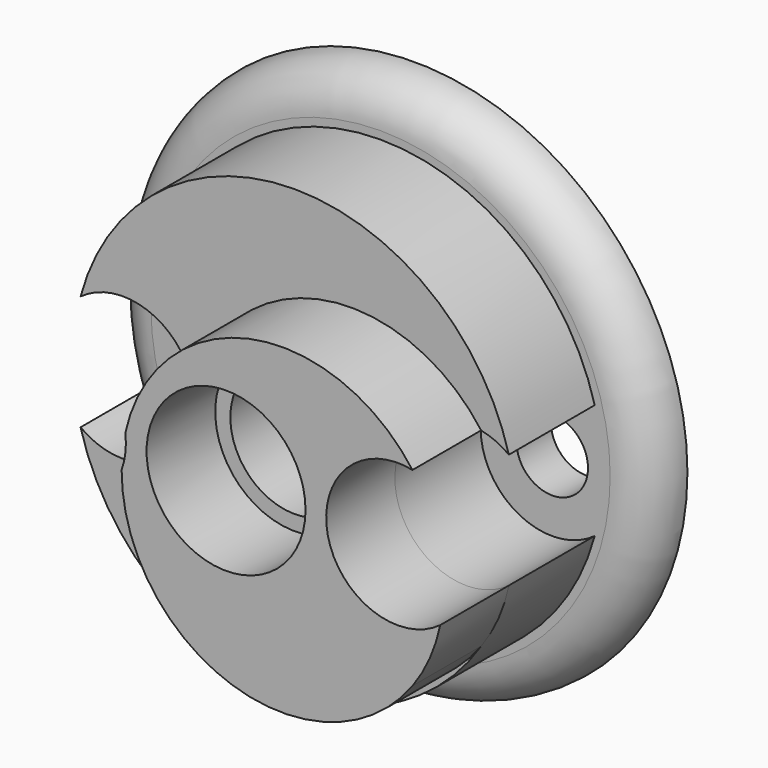
from build123d import *

# Parameters (mm, degrees)
F0_R     = 19.05
F0_R_2   = 2.5
F0_R_3   = 4.5
F1_DEPTH = 3
F2_R     = 2.99999
F3_R     = 4.5
F4_DEPTH = 7.5
F5_R     = 5.555
F6_DEPTH = 6


# Not quite as in the source:
# - a fillet or chamfer is up to 0.001 mm smaller than in the source, because OpenCascade refuses the exact size


with BuildPart() as f1:
    # F0 (on Front) → F1 (new body)
    with BuildSketch(Plane.XZ):
        Circle(F0_R)
        with Locations((-12, 0)):
            Circle(F0_R_2, mode=Mode.SUBTRACT)
        Circle(F0_R_3, mode=Mode.SUBTRACT)
        with Locations((12, 0)):
            Circle(F0_R_2, mode=Mode.SUBTRACT)
    extrude(amount=F1_DEPTH)

    # F2 (radius 3 in the source; OpenCascade refuses exactly that, so slightly less here)
    f2_edges = [f1.edges().sort_by_distance(p)[0] for p in [
        (-19.05, -3, 0),
    ]]
    fillet(f2_edges, radius=F2_R)

    # F3 (on face) → F4 (join)
    with BuildSketch(Plane.XZ.offset(3)):
        with BuildLine():
            ThreePointArc((14.96875, -4.0232478717), (7, 0), (14.96875, 4.0232478717))
            ThreePointArc((14.96875, 4.0232478717), (0, 15.5), (-14.96875, 4.0232478717))
            ThreePointArc((-14.96875, 4.0232478717), (-9.7465304528, 4.4633927678), (-7, 0))
            ThreePointArc((-7, 0), (-9.7465304528, -4.4633927678), (-14.96875, -4.0232478717))
            ThreePointArc((-14.96875, -4.0232478717), (0, -15.5), (14.96875, -4.0232478717))
        make_face()
        Circle(F3_R, mode=Mode.SUBTRACT)
    extrude(amount=F4_DEPTH)

    # F5 (on face) → F6 (join)
    with BuildSketch(Plane.XZ.offset(10.5)):
        with BuildLine():
            ThreePointArc((13.0379586998, -8.3822212416), (14.2369080678, -6.3061863212), (14.96875, -4.0232478717))
            ThreePointArc((14.96875, -4.0232478717), (14.1719474758, -6.2774122648), (13.0379586998, -8.3822212416))
        make_face()
        with BuildLine():
            ThreePointArc((13.0379586998, -8.3822212416), (14.1719474758, -6.2774122648), (14.96875, -4.0232478717))
            ThreePointArc((14.96875, -4.0232478717), (7.1141405648, -1.0622511849), (13.0303045981, 4.8926958249))
            ThreePointArc((13.0303045981, 4.8926958249), (1.6209007027, 9.2560887381), (-7.0415959869, 0.6436067458))
            ThreePointArc((-7.0415959869, 0.6436067458), (-7.0298229821, -0.5452892911), (-7.2990861299, -1.7033522202))
            ThreePointArc((-7.2990861299, -1.7033522202), (0.4406594059, -12.4383718384), (13.0379586998, -8.3822212416))
        make_face()
        Circle(F5_R, mode=Mode.SUBTRACT)
    extrude(amount=F6_DEPTH)


solid = f1.part
